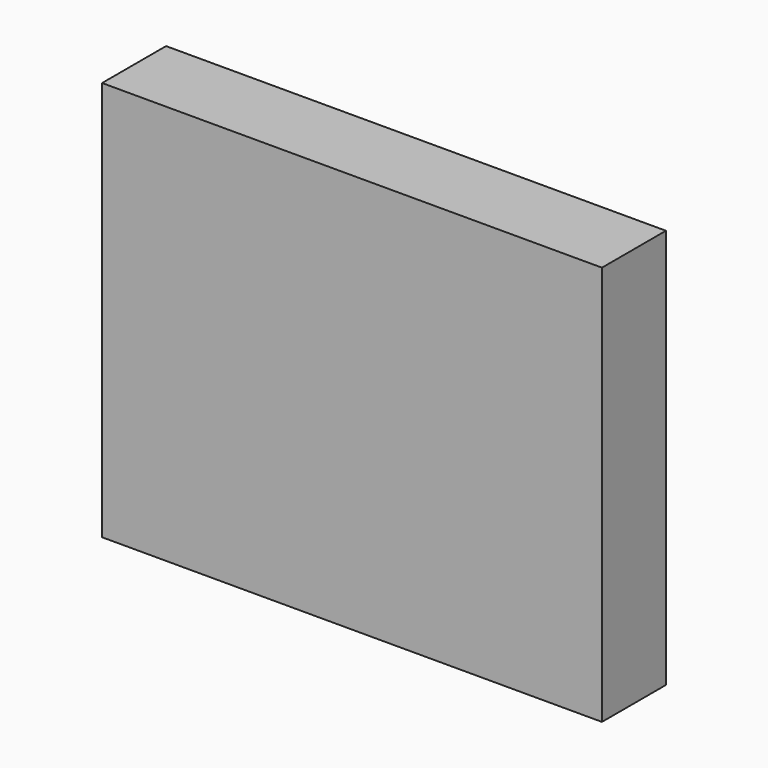
from build123d import *

# Parameters (mm, degrees)
F0_W        = 50
F0_H        = 40
F1_DEPTH    = 8
F2_T        = -1
F3_W        = 15.0767099112
F3_H        = 12.3402951285
F4_DEPTH    = 10
F5_T        = 0.5
F5_T3_DEPTH = 8
F5_T5_DEPTH = 49
F5_T7_DEPTH = 39


# Not quite as in the source:
# - a shell that OpenCascade refuses in one call is made with other operations: the cavity is built on its own and cut out


with BuildPart() as f1:
    # F0 (on Front) → F1 (new body)
    with BuildSketch(Plane.XZ):
        with Locations((-5.8206513731, 0.1503955573)):
            Rectangle(F0_W, F0_H)
    extrude(amount=F1_DEPTH)

    # F2
    f2_openings = [f1.faces().sort_by_distance(p)[0] for p in [
        (-5.820651, 0, 0.150396),
    ]]
    offset(amount=F2_T, openings=f2_openings)

    # F3 (on face) → F4 (join)
    with BuildSketch(Plane(origin=(0, -7, 0), x_dir=(-1, 0, 0), z_dir=(0, 1, 0))):
        with Locations((7.5383549556, -0.1530931331)):
            Rectangle(F3_W, F3_H)
    extrude(amount=F4_DEPTH)

    # F5: shell of thickness 0.5, made by hand


with BuildPart() as f5_core1:
    # F5_t2: copy of F1
    add(f1.part)

    # the walls: a layer under each face that stays
    f5_faces = [f5_core1.faces().sort_by_distance(p)[0] for p in [
        (-5.8206513731, -4, 20.1503955573),
        (19.1793486269, -4, 0.1503955573),
        (-30.8206513731, -4, 0.1503955573),
        (11.3668486269, 0, -19.3557772822),
        (-5.8206513731, -8, 0.1503955573),
        (-5.8206513731, -4, -19.8496044427),
        (-5.8206513731, -3.5, 19.1503955573),
        (18.1793486269, -3.5, 0.1503955573),
        (-5.8206513731, -3.5, -18.8496044427),
        (-29.8206513731, -3.5, 0.1503955573),
        (-21.8206513731, -7, -12.5162711094),
    ]]
    thicken(f5_faces, amount=-F5_T, mode=Mode.SUBTRACT)

    # F5_s4 → F5_t3 (cut)
    with BuildSketch(Plane.XZ.offset(-0.5)):
        Polygon((18.1743486269, 19.1453955573), (18.1793486269, 19.6503955573), (18.6793486269, 19.6503955573), (18.6793486269, 19.1503955573), align=None)
        Polygon((-29.8156513731, 19.1453955573), (-29.8206513731, 19.6503955573), (-30.3206513731, 19.6503955573), (-30.3206513731, 19.1503955573), align=None)
        Polygon((18.1743486269, -18.8446044427), (18.6793486269, -18.8496044427), (18.6793486269, -19.3496044427), (18.1793486269, -19.3496044427), align=None)
        Polygon((-29.8156513731, -18.8446044427), (-29.8206513731, -19.3496044427), (-30.3206513731, -19.3496044427), (-30.3206513731, -18.8496044427), align=None)
    extrude(amount=F5_T3_DEPTH, mode=Mode.SUBTRACT)

    # F5_s6 → F5_t5 (cut)
    with BuildSketch(Plane.YZ.offset(-30.3206513731)):
        Polygon((-6.995, 19.1453955573), (-7, 19.6503955573), (-7.5, 19.6503955573), (-7.5, 19.1503955573), align=None)
        Polygon((-6.995, -18.8446044427), (-7, -19.3496044427), (-7.5, -19.3496044427), (-7.5, -18.8496044427), align=None)
    extrude(amount=F5_T5_DEPTH, mode=Mode.SUBTRACT)

    # F5_s8 → F5_t7 (cut)
    with BuildSketch(Plane.XY.offset(-19.3496044427)):
        Polygon((18.1743486269, -6.995), (18.6793486269, -7), (18.6793486269, -7.5), (18.1793486269, -7.5), align=None)
        Polygon((-29.8156513731, -6.995), (-30.3206513731, -7), (-30.3206513731, -7.5), (-29.8206513731, -7.5), align=None)
    extrude(amount=F5_T7_DEPTH, mode=Mode.SUBTRACT)


with BuildPart() as f1_1:
    add(f1.part)

    # what is left inside the walls is the cavity
    f5_cavity = [f5_core1.part.solids().sort_by_distance(p)[0] for p in [
        (-7.538355, -7.495, -2.209809),
    ]]
    add(f5_cavity, mode=Mode.SUBTRACT)


solid = f1_1.part
